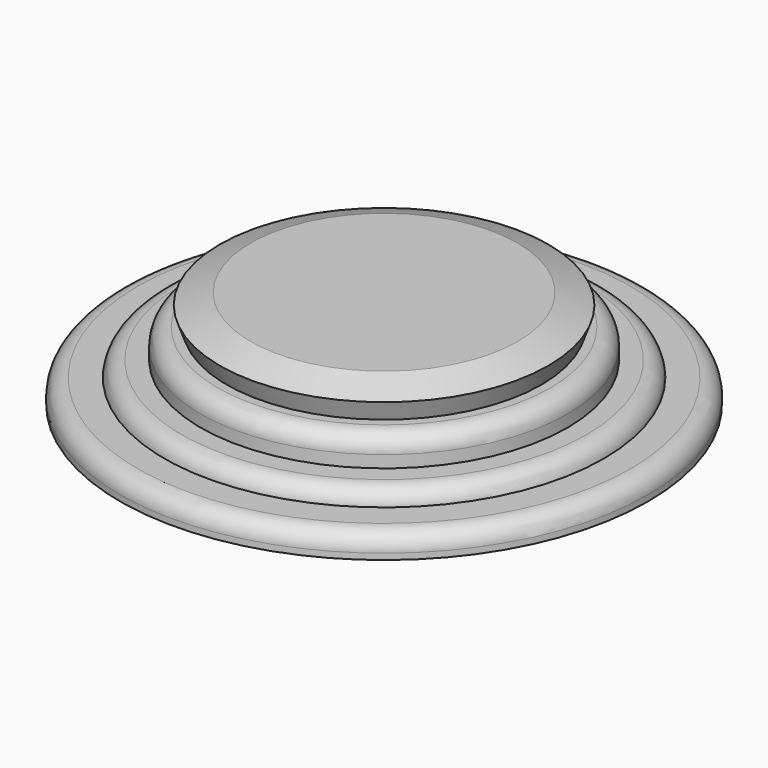
from build123d import *

# Parameters (mm, degrees)
F0_R      = 77.7501635543
F0_R_2    = 64.6980648952
F1_DEPTH  = 6.858
F0_R_3    = 54.0479242204
F2_DEPTH  = 11.43
F0_R_4    = 39.0523448649
F3_DEPTH  = 20.066
F5_DEPTH  = 25.654
F5_TAPER  = -20
F5_FACE_R = 48.3896372547
F6_DEPTH  = 3.302
F6_TAPER  = 70


# Not quite as in the source:
# - a fillet or chamfer that OpenCascade refuses, or shapes differently, is made with other operations: its cross-section is extruded or revolved along the edge and cut away or added


with BuildPart() as f1:
    # F0 (on Top) → F1 (new body)
    with BuildSketch(Plane.XY):
        Circle(F0_R)
        Circle(F0_R_2, mode=Mode.SUBTRACT)
    extrude(amount=F1_DEPTH)

    # F0 (on Top) → F2 (join)
    with BuildSketch(Plane.XY):
        Circle(F0_R_2)
        Circle(F0_R_3, mode=Mode.SUBTRACT)
    extrude(amount=F2_DEPTH)

    # F0 (on Top) → F3 (join)
    with BuildSketch(Plane.XY):
        Circle(F0_R_3)
        Circle(F0_R_4, mode=Mode.SUBTRACT)
    extrude(amount=F3_DEPTH)

    # F4: fillet of radius 5.08 on 3 edges, made by hand

    # F4_s1 → F4_t2 (revolve, cut)
    with BuildSketch(Plane.XZ):
        with BuildLine():
            ThreePointArc((48.9679242204, 20.066), (52.5600266688, 18.5781024484), (54.0479242204, 14.986))
            Line((54.0479242204, 14.986), (54.0479242204, 20.066))
            Line((54.0479242204, 20.066), (48.9679242204, 20.066))
        make_face()
    revolve(axis=Axis((0, 0, 20.066), (0, 0, 1)), mode=Mode.SUBTRACT)

    # F4_s3 → F4_t4 (revolve, cut)
    with BuildSketch(Plane.XZ):
        with BuildLine():
            ThreePointArc((64.6980648952, 6.858), (63.0512963124, 10.1174288314), (59.6435287147, 11.43))
            Line((59.6435287147, 11.43), (64.6980648952, 11.43))
            Line((64.6980648952, 11.43), (64.6980648952, 6.858))
        make_face()
    revolve(axis=Axis((0, 0, 11.43), (0, 0, 1)), mode=Mode.SUBTRACT)

    # F4_s5 → F4_t6 (revolve, cut)
    with BuildSketch(Plane.XZ):
        with BuildLine():
            ThreePointArc((77.7501635543, 1.778), (76.2622660027, 5.3701024484), (72.6701635543, 6.858))
            Line((72.6701635543, 6.858), (77.7501635543, 6.858))
            Line((77.7501635543, 6.858), (77.7501635543, 1.778))
        make_face()
    revolve(axis=Axis((0, 0, 6.858), (0, 0, 1)), mode=Mode.SUBTRACT)

    # F0 (on Top) → F5 (join)
    with BuildSketch(Plane.XY):
        Circle(F0_R_4)
    extrude(amount=F5_DEPTH, taper=F5_TAPER)

    # F5_face (on face) → F6 (join)
    with BuildSketch(Plane.XY.offset(25.654)):
        Circle(F5_FACE_R)
    extrude(amount=F6_DEPTH, taper=F6_TAPER)


solid = f1.part
